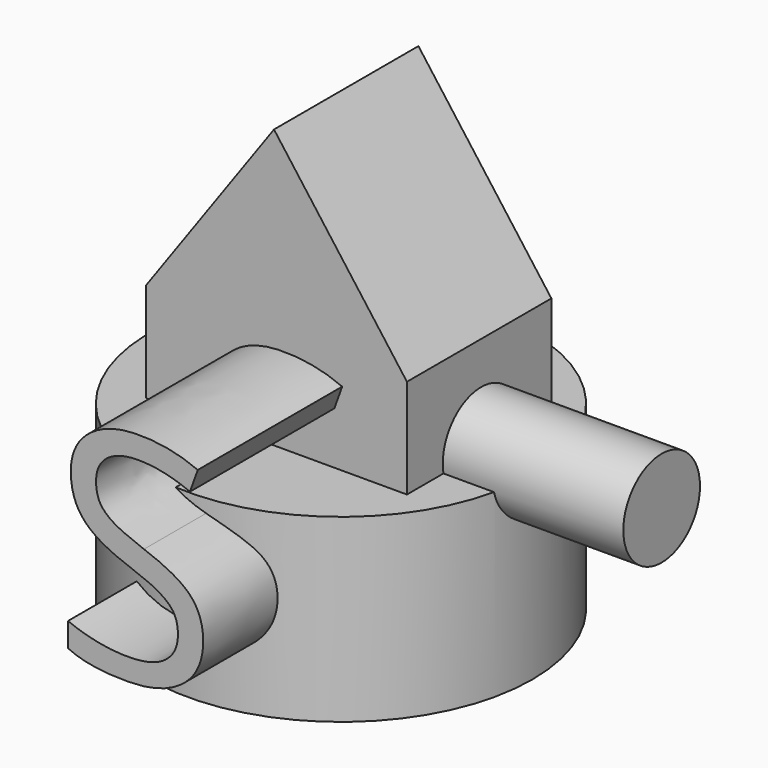
from build123d import *

# Parameters (mm, degrees)
F0_W         = 36.7145463824
F0_H         = 39.3700003624
F1_DEPTH     = 25.4
F2_TEXT_SIZE = 42.3333323043
F3_DEPTH     = 25.4
F5_DEPTH     = 25.4
F4_R         = 6.7439684478
F6_DEPTH     = 25.4
F7_R         = 26.938295065
F8_DEPTH     = 25.4


# Not quite as in the source:
# - Text() gives the source's letters only with a copy of the font that has no kerning and outlines rounded to 1/6400 em; it was checked with that copy


with BuildPart() as f1:
    # F0 (on Front) → F1 (new body)
    with BuildSketch(Plane.XZ):
        Polygon((18.0109106004, 64.5390897989), (0, 39.3700003624), (36.7145463824, 39.3700003624), align=None)
        with Locations((18.3572731912, 19.6850001812)):
            Rectangle(F0_W, F0_H)
    extrude(amount=F1_DEPTH)

    # F2 (on face) → F3 (join)
    with BuildSketch(Plane.XZ.offset(25.4)):
        with Locations((7.1581806988, 6.811818108)):
            Text('S', F2_TEXT_SIZE, font='Open Sans', text_align=(TextAlign.LEFT, TextAlign.BOTTOM))
    extrude(amount=F3_DEPTH)

    # F5 (cut): a face of the model
    f5_faces = [f1.faces().sort_by_distance(p)[0] for p in [
        (9.0054553002, -12.7, 51.9545450807),
    ]]
    extrude(f5_faces, amount=F5_DEPTH, mode=Mode.SUBTRACT)

    # F4 (on face) → F6 (join)
    with BuildSketch(Plane.YZ.offset(36.7145463824)):
        with Locations((-12.3536363244, 26.6700014472)):
            Circle(F4_R)
    extrude(amount=F6_DEPTH)

    # F7 (on Top) → F8 (join)
    with BuildSketch(Plane.XY):
        with Locations((17.5490900874, -13.0463633686)):
            Circle(F7_R)
    extrude(amount=F8_DEPTH)


solid = f1.part
